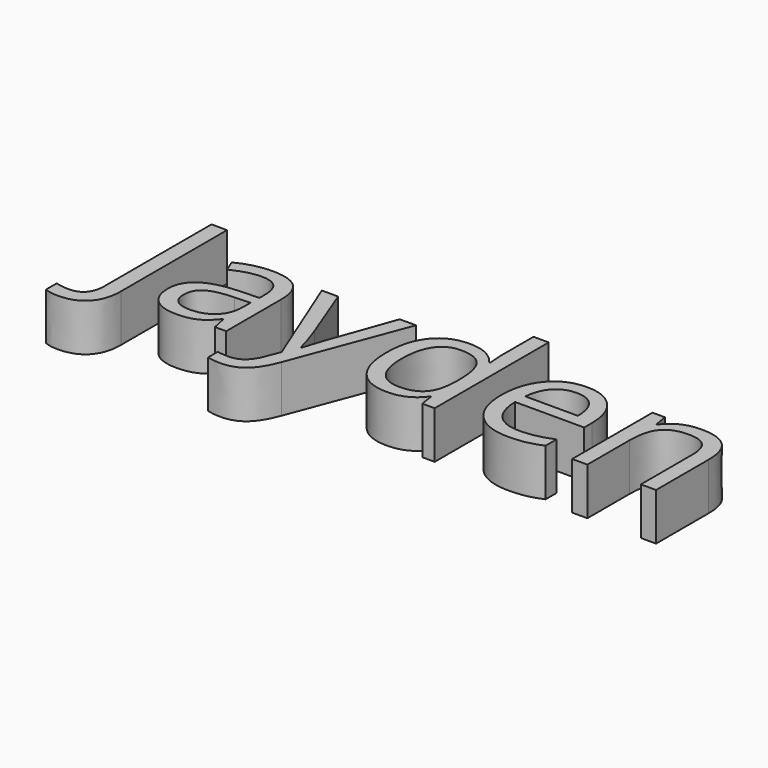
from build123d import *

# Parameters (mm, degrees)
F0_TEXT_SIZE = 100.8587294362
F1_DEPTH     = 25.4


# Not quite as in the source:
# - Text() gives the source's letters only with a copy of the font that has no kerning and outlines rounded to 1/6400 em; it was checked with that copy


with BuildPart() as f1:
    # F0 (on Top) → F1 (new body)
    with BuildSketch(Plane.XY):
        with Locations((-148.1518875808, -33.6137168342)):
            Text('Jayden', F0_TEXT_SIZE, font='Open Sans', text_align=(TextAlign.LEFT, TextAlign.BOTTOM))
    extrude(amount=F1_DEPTH)


solid = f1.part
